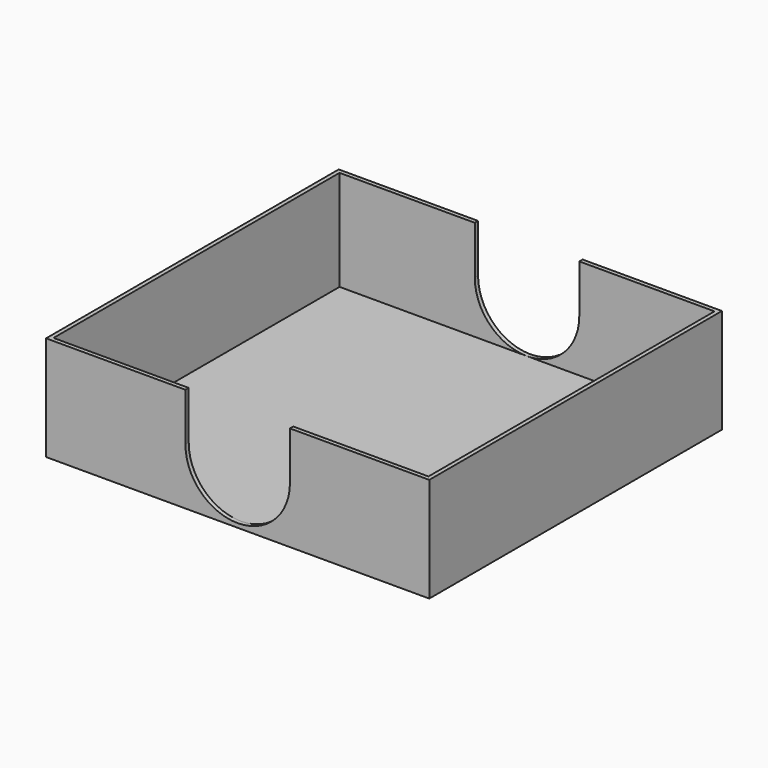
from build123d import *

# Parameters (mm, degrees)
F0_W     = 139.7
F0_H     = 133.35
F1_DEPTH = 38.1
F2_T     = -1.5
F4_DEPTH = 1.5


# Not quite as in the source:
# - a pattern or mirror of a feature is missing from the dataset's text; its kind, count and spacing are read off the source's solid


with BuildPart() as f1:
    # F0 (on Top) → F1 (new body)
    with BuildSketch(Plane.XY):
        Rectangle(F0_W, F0_H)
    extrude(amount=F1_DEPTH)

    # F2
    f2_openings = [f1.faces().sort_by_distance(p)[0] for p in [
        (0, 0, 38.1),
    ]]
    offset(amount=F2_T, openings=f2_openings)

    # F3 (on face) → F4 (cut)
    with BuildSketch(Plane.XZ.offset(66.675)):
        with BuildLine():
            Line((19.05, 20.55), (-19.05, 20.55))
            ThreePointArc((-19.05, 20.55), (0, 1.5), (19.05, 20.55))
        make_face()
        with BuildLine():
            Line((-19.05, 38.1), (-19.05, 20.55))
            ThreePointArc((-19.05, 20.55), (-15.8753360228, 31.0797771184), (-7.4094534211, 38.1))
            Line((-7.4094534211, 38.1), (-19.05, 38.1))
        make_face()
        with BuildLine():
            ThreePointArc((-7.4094534211, 38.1), (-15.8753360228, 31.0797771184), (-19.05, 20.55))
            Line((-19.05, 20.55), (19.05, 20.55))
            ThreePointArc((19.05, 20.55), (15.8753360228, 31.0797771184), (7.4094534211, 38.1))
            Line((7.4094534211, 38.1), (-7.4094534211, 38.1))
        make_face()
        with BuildLine():
            ThreePointArc((7.4094534211, 38.1), (15.8753360228, 31.0797771184), (19.05, 20.55))
            Line((19.05, 20.55), (19.05, 38.1))
            Line((19.05, 38.1), (7.4094534211, 38.1))
        make_face()
        with BuildLine():
            ThreePointArc((7.4094534211, 38.1), (0, 39.6), (-7.4094534211, 38.1))
            Line((-7.4094534211, 38.1), (7.4094534211, 38.1))
        make_face()
    f4 = extrude(amount=-F4_DEPTH, mode=Mode.SUBTRACT)

    # F4_copies: F4 across plane
    add(f4.mirror(Plane.ZX), mode=Mode.SUBTRACT)


solid = f1.part
